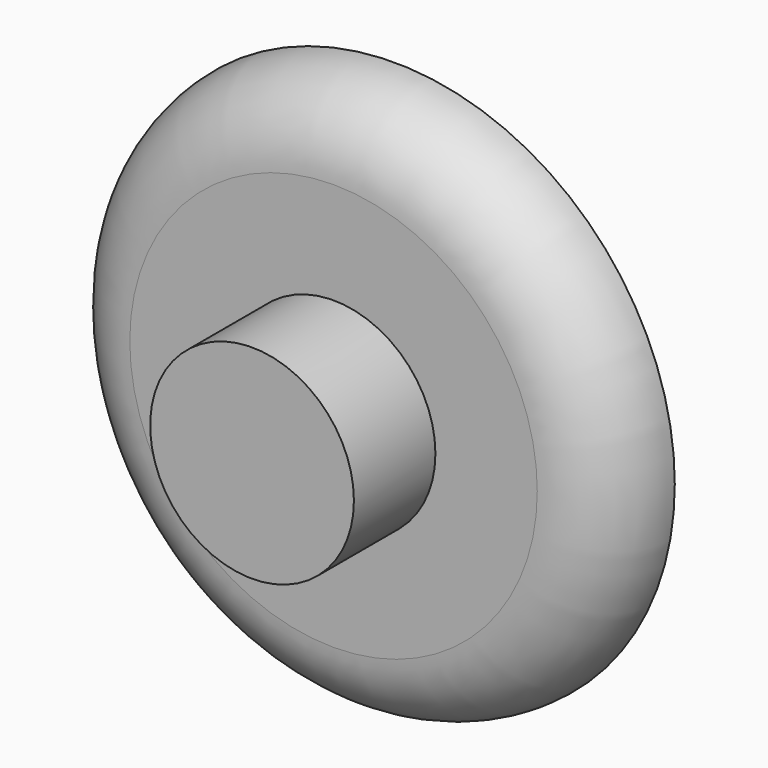
from build123d import *

# Parameters (mm, degrees)
F2_R     = 4
F3_DEPTH = 4
F4_R     = 2.99999


# Not quite as in the source:
# - a fillet or chamfer is up to 0.001 mm smaller than in the source, because OpenCascade refuses the exact size


with BuildPart() as f1:
    # F0 (on Top) → F1 (revolve)
    with BuildSketch(Plane.XY):
        with BuildLine():
            ThreePointArc((11, 1), (5.5339321669, 0.1267461642), (0, 0))
            Line((0, 0), (0, -2))
            Line((0, -2), (11, -2))
            Line((11, -2), (11, 1))
        make_face()
    revolve(axis=Axis((0, -1, 0), (0, -1, 0)))

    # F2 (on face) → F3 (join)
    with BuildSketch(Plane.XZ.offset(2)):
        Circle(F2_R)
    extrude(amount=F3_DEPTH)

    # F4 (radius 3 in the source; OpenCascade refuses exactly that, so slightly less here)
    f4_edges = [f1.edges().sort_by_distance(p)[0] for p in [
        (-11, -2, 0),
    ]]
    fillet(f4_edges, radius=F4_R)


solid = f1.part
